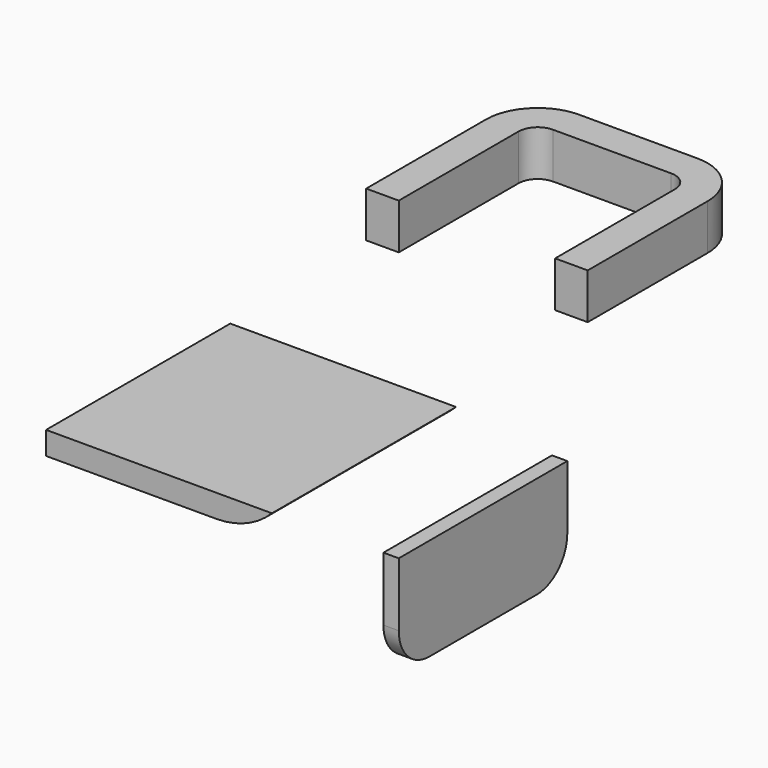
from build123d import *

# Parameters (mm, degrees)
F1_W        = 4.31708619
F1_H        = 6.0439207591
F3_W        = 29.9317967147
F3_H        = 30.5074118078
F4_DEPTH    = 3.048
F5_T1_DEPTH = 67.3373928333
F7_DEPTH    = 2.032


# Not quite as in the source:
# - a fillet or chamfer that OpenCascade refuses, or shapes differently, is made with other operations: its cross-section is extruded or revolved along the edge and cut away or added


with BuildPart() as f2:
    # F2: sweep along a path in F0
    with BuildLine(Plane.XY) as f2_path:
        Line((0, 0), (0, 19.8403237551))
        ThreePointArc((0, 19.8403237551), (0.7439487758, 21.6363749794), (2.54, 22.3803237551))
        Line((2.54, 22.3803237551), (18.1820148295, 22.3803237551))
        ThreePointArc((18.1820148295, 22.3803237551), (19.9780660537, 21.6363749794), (20.7220148295, 19.8403237551))
        Line((20.7220148295, 19.8403237551), (20.7220148295, 0))
    # F1 (on Front) → F2 (sweep)
    with BuildSketch(Plane.XZ):
        with Locations((-2.158543095, 3.0219603796)):
            Rectangle(F1_W, F1_H)
    sweep(path=f2_path.line)


with BuildPart() as f4:
    # F3 (on Top) → F4 (new body)
    with BuildSketch(Plane.XY):
        with Locations((14.9658983573, -43.1708637625)):
            Rectangle(F3_W, F3_H)
    extrude(amount=F4_DEPTH)

    # F5: fillet of radius 10.4245741623 on 1 edges, made by hand

    # F5_s2 → F5_t1 (cut)
    with BuildSketch(Plane.XZ.offset(9.5021673459)):
        with BuildLine():
            ThreePointArc((29.9317967147, 3.048), (26.5516568822, 0.792092891), (22.5658005096, 0))
            Line((22.5658005096, 0), (29.9317967147, 0))
            Line((29.9317967147, 0), (29.9317967147, 3.048))
        make_face()
    extrude(amount=F5_T1_DEPTH, mode=Mode.SUBTRACT)


with BuildPart() as f7:
    # F6 (on Right) → F7 (new body)
    with BuildSketch(Plane.YZ):
        with BuildLine():
            ThreePointArc((0, -44.1347840559), (1.4878975516, -47.7268865044), (5.08, -49.2147840559))
            Line((5.08, -49.2147840559), (22.837155996, -49.2147840559))
            ThreePointArc((22.837155996, -49.2147840559), (26.4292584444, -47.7268865044), (27.917155996, -44.1347840559))
            Line((27.917155996, -44.1347840559), (27.917155996, -35.6879122555))
            Line((27.917155996, -35.6879122555), (0, -35.6879122555))
            Line((0, -35.6879122555), (0, -44.1347840559))
        make_face()
    extrude(amount=-F7_DEPTH)


solid = Compound([f2.part, f4.part, f7.part])
